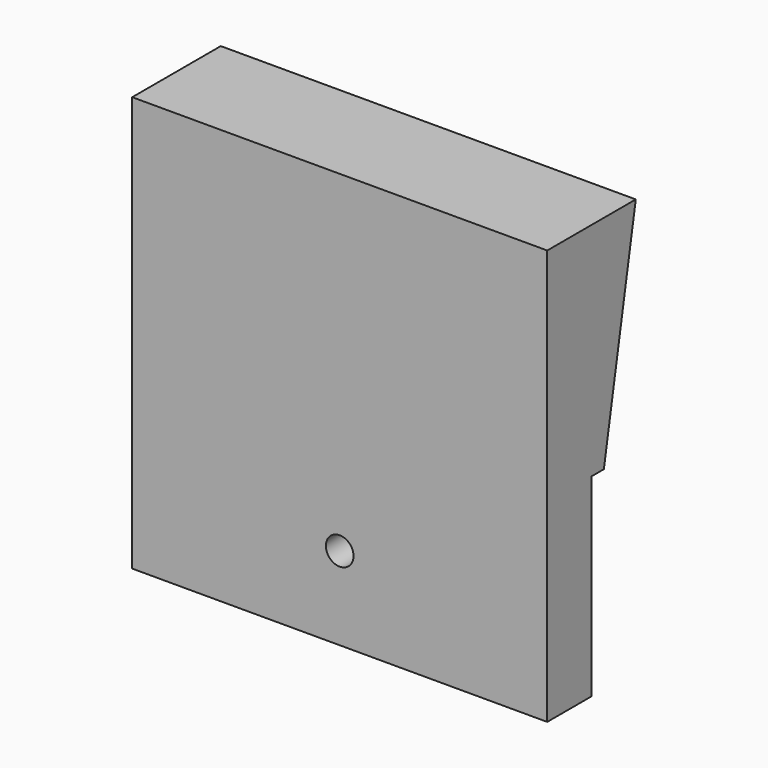
from build123d import *

# Parameters (mm, degrees)
F0_W     = 150
F0_H     = 150
F1_DEPTH = 20
F2_W     = 150
F2_H     = 80
F3_DEPTH = 20
F5_DEPTH = 150.001
F6_R     = 5
F7_DEPTH = 40.001


# Not quite as in the source:
# - a feature names something its author has since deleted; it is built from what else it names


with BuildPart() as f1:
    # F0 (on Front) → F1 (new body)
    with BuildSketch(Plane.XZ):
        Rectangle(F0_W, F0_H)
    extrude(amount=F1_DEPTH)

    # F2 (on face) → F3 (join)
    with BuildSketch(Plane(origin=(0, 0, 0), x_dir=(-1, 0, 0), z_dir=(0, 1, 0))):
        with Locations((0, 35)):
            Rectangle(F2_W, F2_H)
    extrude(amount=F3_DEPTH)

    # F4 (on face) → F5 (cut, through all)
    with BuildSketch(Plane.YZ.offset(75)):
        Polygon((20, -5), (20, 75), (5.5873245001, -5), align=None)
    extrude(amount=-F5_DEPTH, mode=Mode.SUBTRACT)

    # F6 (on face) → F7 (cut, through all)
    with BuildSketch(Plane.XZ.offset(20)):
        with Locations((0, -45)):
            Circle(F6_R)
    extrude(amount=-F7_DEPTH, mode=Mode.SUBTRACT)


solid = f1.part
